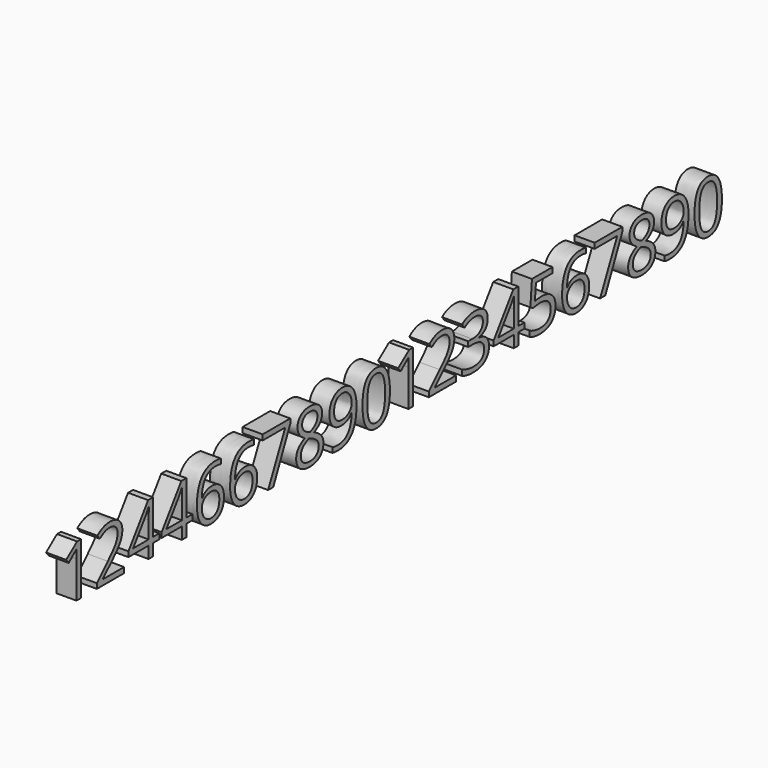
from build123d import *

# Parameters (mm, degrees)
F0_TEXT_SIZE = 90.4227710432
F1_DEPTH     = 25


# Not quite as in the source:
# - Text() gives the source's letters only with a copy of the font that has no kerning and outlines rounded to 1/6400 em; it was checked with that copy


with BuildPart() as f1:
    # F0 (on Right) → F1 (new body)
    with BuildSketch(Plane.YZ):
        with Locations((0, 0)):
            Text('12446678901234567890', F0_TEXT_SIZE, font='Open Sans', text_align=(TextAlign.LEFT, TextAlign.BOTTOM))
    extrude(amount=F1_DEPTH)


solid = f1.part
